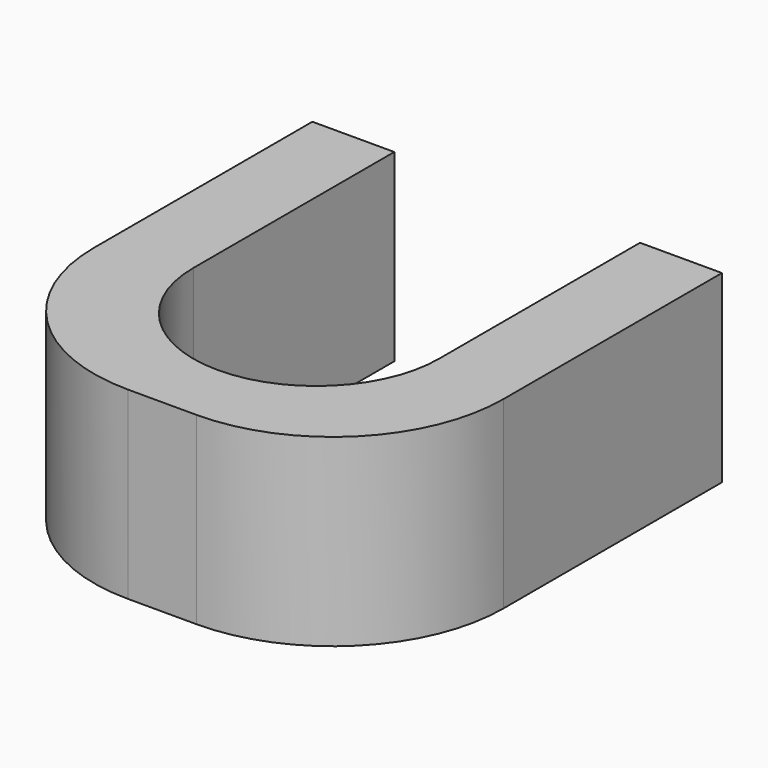
from build123d import *

# Parameters (mm, degrees)
F1_DEPTH = 6.858
F2_R     = 4.57199
F3_R     = 6.35


# Not quite as in the source:
# - a fillet or chamfer is up to 0.001 mm smaller than in the source, because OpenCascade refuses the exact size


with BuildPart() as f1:
    # F0 (on Top) → F1 (new body)
    with BuildSketch(Plane.XY):
        Polygon((-7.62, -8.255), (7.62, -8.255), (7.62, 8.255), (4.572, 8.255), (4.572, -5.6657525711), (-4.572, -5.6657525711), (-4.572, 8.255), (-7.62, 8.255), align=None)
    extrude(amount=F1_DEPTH)

    # F2 (radius 4.572 in the source; OpenCascade refuses exactly that, so slightly less here)
    f2_edges = [f1.edges().sort_by_distance(p)[0] for p in [
        (-4.572, -5.665753, 3.429),
        (4.572, -5.665753, 3.429),
    ]]
    fillet(f2_edges, radius=F2_R)

    # F3
    f3_edges = [f1.edges().sort_by_distance(p)[0] for p in [
        (7.62, -8.255, 3.429),
        (-7.62, -8.255, 3.429),
    ]]
    fillet(f3_edges, radius=F3_R)


solid = f1.part
